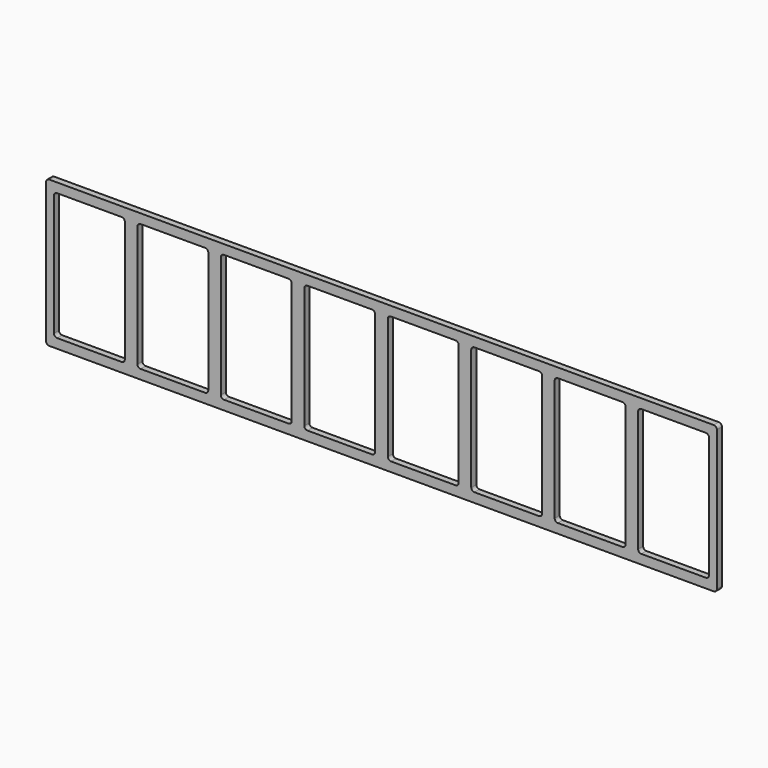
from build123d import *

# Parameters (mm, degrees)
F0_W     = 213
F0_H     = 46.5
F0_W_2   = 22.5
F0_H_2   = 40.5
F1_DEPTH = 2
F2_R     = 1


# Not quite as in the source:
# - a feature names something its author has since deleted; it is built from what else it names


with BuildPart() as f1:
    # F0 (on Front) → F1 (new body)
    with BuildSketch(Plane.XZ):
        with Locations((1.4150981574, 5.1332409506)):
            Rectangle(F0_W, F0_H)
        with Locations((-91.3349018426, 5.1332409506)):
            Rectangle(F0_W_2, F0_H_2, mode=Mode.SUBTRACT)
        with Locations((-64.8349018426, 5.1332409506)):
            Rectangle(F0_W_2, F0_H_2, mode=Mode.SUBTRACT)
        with Locations((-38.3349018426, 5.1332409506)):
            Rectangle(F0_W_2, F0_H_2, mode=Mode.SUBTRACT)
        with Locations((-11.8349018426, 5.1332409506)):
            Rectangle(F0_W_2, F0_H_2, mode=Mode.SUBTRACT)
        with Locations((14.6650981574, 5.1332409506)):
            Rectangle(F0_W_2, F0_H_2, mode=Mode.SUBTRACT)
        with Locations((41.1650981574, 5.1332409506)):
            Rectangle(F0_W_2, F0_H_2, mode=Mode.SUBTRACT)
        with Locations((67.6650981574, 5.1332409506)):
            Rectangle(F0_W_2, F0_H_2, mode=Mode.SUBTRACT)
        with Locations((94.1650981574, 5.1332409506)):
            Rectangle(F0_W_2, F0_H_2, mode=Mode.SUBTRACT)
    extrude(amount=F1_DEPTH)

    # F2
    f2_edges = [f1.edges().sort_by_distance(p)[0] for p in [
        (-80.084902, -1, 25.383241),
        (-102.584902, -1, 25.383241),
        (-80.084902, -1, -15.116759),
        (-102.584902, -1, -15.116759),
        (107.915098, -1, 28.383241),
        (107.915098, -1, -18.116759),
        (-105.084902, -1, 28.383241),
        (-105.084902, -1, -18.116759),
        (-76.084902, -1, 25.383241),
        (-49.584902, -1, 25.383241),
        (-23.084902, -1, 25.383241),
        (3.415098, -1, 25.383241),
        (29.915098, -1, 25.383241),
        (56.415098, -1, 25.383241),
        (82.915098, -1, 25.383241),
        (-53.584902, -1, 25.383241),
        (-27.084902, -1, 25.383241),
        (-0.584902, -1, 25.383241),
        (25.915098, -1, 25.383241),
        (52.415098, -1, 25.383241),
        (78.915098, -1, 25.383241),
        (105.415098, -1, 25.383241),
        (-76.084902, -1, -15.116759),
        (-49.584902, -1, -15.116759),
        (-23.084902, -1, -15.116759),
        (3.415098, -1, -15.116759),
        (29.915098, -1, -15.116759),
        (56.415098, -1, -15.116759),
        (82.915098, -1, -15.116759),
        (-53.584902, -1, -15.116759),
        (-27.084902, -1, -15.116759),
        (-0.584902, -1, -15.116759),
        (25.915098, -1, -15.116759),
        (52.415098, -1, -15.116759),
        (78.915098, -1, -15.116759),
        (105.415098, -1, -15.116759),
    ]]
    fillet(f2_edges, radius=F2_R)


solid = f1.part
